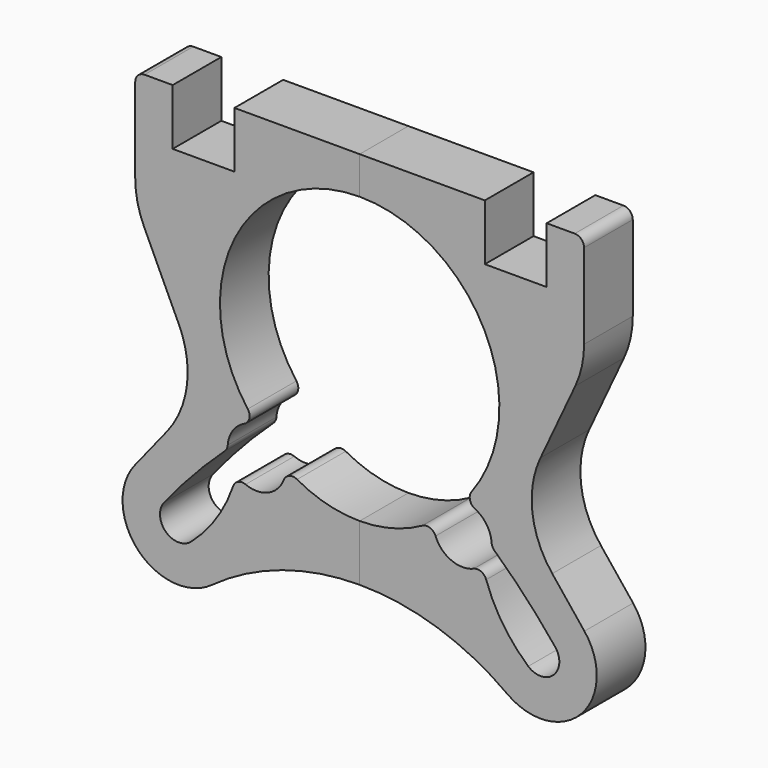
from build123d import *
from build123d import SkipClean  # not in build123d's __all__

# Parameters (mm, degrees)
F2_DEPTH = 1.625
F3_R     = 0.5
F4_R     = 5


with BuildPart() as f2:
    # F1 (on Front) → F2 (new body, symmetric)
    with BuildSketch(Plane.XZ):
        with BuildLine():
            ThreePointArc((0, -6.875), (-2.0724417463, -6.5551971906), (-3.9520768911, -5.6255411515))
            ThreePointArc((-3.9520768911, -5.6255411515), (-4.8570002775, -7.1160909953), (-6.5757097792, -6.8217054979))
            ThreePointArc((-6.5757097792, -6.8217054979), (-7.4894639741, -8.9857797177), (-9.0066893746, -10.7791539234))
            ThreePointArc((-9.0066893746, -10.7791539234), (-10.3561219729, -10.7473840389), (-10.4445927673, -9.400479966))
            ThreePointArc((-10.4445927673, -9.400479966), (-8.8177667586, -7.5260240462), (-7.0479231089, -5.7859661986))
            ThreePointArc((-7.0479231089, -5.7859661986), (-6.6159518229, -4.6300438958), (-5.4766665535, -4.1559293139))
            ThreePointArc((-5.4766665535, -4.1559293139), (-6.837727437, 3.9011833784), (0, 8.375))
            Line((0, 8.375), (0, 10.375))
            Line((0, 10.375), (-6.6871520114, 10.375))
            Line((-6.6871520114, 10.375), (-6.6871520114, 7.375))
            Line((-6.6871520114, 7.375), (-9.9871520114, 7.375))
            Line((-9.9871520114, 7.375), (-9.9871520114, 10.375))
            Line((-9.9871520114, 10.375), (-11.9871520114, 10.375))
            Line((-11.9871520114, 10.375), (-11.9871520114, 4.2244328171))
            Line((-11.9871520114, 4.2244328171), (-8.5746230978, -3.0885299193))
            ThreePointArc((-8.5746230978, -3.0885299193), (-8.458137965, -3.3292198832), (-8.3348983214, -3.5665222959))
            Line((-8.3348983214, -3.5665222959), (-12.0057025921, -8.1503055323))
            ThreePointArc((-12.0057025921, -8.1503055323), (-11.8324993376, -12.098674705), (-7.8959026306, -12.4491384793))
            ThreePointArc((-7.8959026306, -12.4491384793), (-4.1524531082, -10.534781214), (0, -9.875))
            Line((0, -9.875), (0, -6.875))
        make_face()
    extrude(amount=F2_DEPTH, both=True)

    # F3
    f3_edges = [f2.edges().sort_by_distance(p)[0] for p in [
        (-3.952077, 0, -5.625541),
        (-7.047923, 0, -5.785966),
        (-11.987152, 0, 10.375),
        (-5.476667, 0, -4.155929),
        (-6.57571, 0, -6.821705),
    ]]
    fillet(f3_edges, radius=F3_R)

    # F4
    f4_edges = [f2.edges().sort_by_distance(p)[0] for p in [
        (-8.334898, 0, -3.566522),
        (-11.987152, 0, 4.224433),
    ]]
    fillet(f4_edges, radius=F4_R)

    # F5: F2 across plane


with BuildPart() as f2_1:
    add(f2.part, clean=False)
    with SkipClean():  # cleaning this boolean's faces spoils the solid; the shape is the same uncleaned
        add(f2.part.mirror(Plane.YZ), clean=False)


solid = f2_1.part
